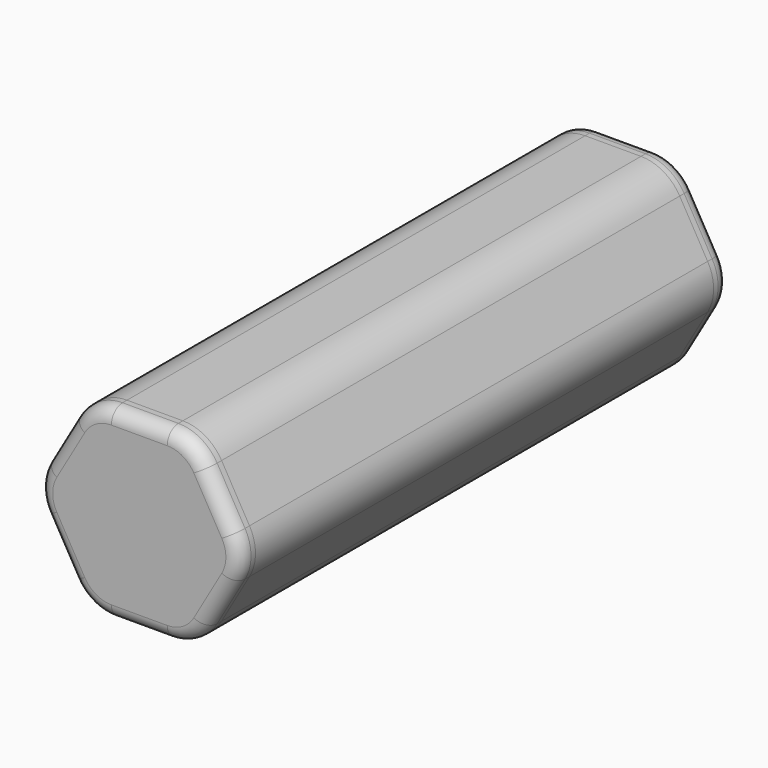
from build123d import *

# Parameters (mm, degrees)
F2_DEPTH = 205
F4_DEPTH = 5
F6_DEPTH = 2
F7_R     = 5
F8_R     = 4.99999


# Not quite as in the source:
# - a fillet or chamfer is up to 0.001 mm smaller than in the source, because OpenCascade refuses the exact size


with BuildPart() as f2:
    # F1 (on Front) → F2 (new body)
    with BuildSketch(Plane.XZ):
        with BuildLine():
            Line((30, 33.3205085668), (10, 33.3205085668))
            ThreePointArc((10, 33.3205085668), (1.9999997545, 31.1769149615), (-3.8564068859, 25.3205083212))
            Line((-3.8564068859, 25.3205083212), (-13.8564068859, 8.0000002455))
            ThreePointArc((-13.8564068859, 8.0000002455), (-16.0000004911, 0), (-13.8564068859, -8.0000002455))
            Line((-13.8564068859, -8.0000002455), (-3.8564068859, -25.3205083212))
            ThreePointArc((-3.8564068859, -25.3205083212), (1.9999997545, -31.1769149615), (10, -33.3205085668))
            Line((10, -33.3205085668), (30, -33.3205085668))
            ThreePointArc((30, -33.3205085668), (38.0000002455, -31.1769149615), (43.8564068859, -25.3205083212))
            Line((43.8564068859, -25.3205083212), (53.8564068859, -8.0000002455))
            ThreePointArc((53.8564068859, -8.0000002455), (56.0000004911, 0), (53.8564068859, 8.0000002455))
            Line((53.8564068859, 8.0000002455), (43.8564068859, 25.3205083212))
            ThreePointArc((43.8564068859, 25.3205083212), (38.0000002455, 31.1769149615), (30, 33.3205085668))
        make_face()
        with BuildLine():
            ThreePointArc((-2.1243560783, 24.3205083212), (2.9999997545, 29.444864154), (10, 31.3205085668))
            Line((10, 31.3205085668), (30, 31.3205085668))
            ThreePointArc((30, 31.3205085668), (37.0000002455, 29.444864154), (42.1243560783, 24.3205083212))
            Line((42.1243560783, 24.3205083212), (52.1243560783, 7.0000002455))
            ThreePointArc((52.1243560783, 7.0000002455), (54.0000004911, 0), (52.1243560783, -7.0000002455))
            Line((52.1243560783, -7.0000002455), (42.1243560783, -24.3205083212))
            ThreePointArc((42.1243560783, -24.3205083212), (37.0000002455, -29.444864154), (30, -31.3205085668))
            Line((30, -31.3205085668), (10, -31.3205085668))
            ThreePointArc((10, -31.3205085668), (2.9999997545, -29.444864154), (-2.1243560783, -24.3205083212))
            Line((-2.1243560783, -24.3205083212), (-12.1243560783, -7.0000002455))
            ThreePointArc((-12.1243560783, -7.0000002455), (-14.0000004911, 0), (-12.1243560783, 7.0000002455))
            Line((-12.1243560783, 7.0000002455), (-2.1243560783, 24.3205083212))
        make_face(mode=Mode.SUBTRACT)
    extrude(amount=F2_DEPTH)


with BuildPart() as f4:
    # F3 (on face) → F4 (new body)
    with BuildSketch(Plane.XZ.offset(205)):
        with BuildLine():
            ThreePointArc((-3.8564068859, -25.3205083212), (1.9999997545, -31.1769149615), (10, -33.3205085668))
            Line((10, -33.3205085668), (30, -33.3205085668))
            ThreePointArc((30, -33.3205085668), (38.0000002455, -31.1769149615), (43.8564068859, -25.3205083212))
            Line((43.8564068859, -25.3205083212), (53.8564068859, -8.0000002455))
            ThreePointArc((53.8564068859, -8.0000002455), (56.0000004911, 0), (53.8564068859, 8.0000002455))
            Line((53.8564068859, 8.0000002455), (43.8564068859, 25.3205083212))
            ThreePointArc((43.8564068859, 25.3205083212), (38.0000002455, 31.1769149615), (30, 33.3205085668))
            Line((30, 33.3205085668), (10, 33.3205085668))
            ThreePointArc((10, 33.3205085668), (1.9999997545, 31.1769149615), (-3.8564068859, 25.3205083212))
            Line((-3.8564068859, 25.3205083212), (-13.8564068859, 8.0000002455))
            ThreePointArc((-13.8564068859, 8.0000002455), (-16.0000004911, 0), (-13.8564068859, -8.0000002455))
            Line((-13.8564068859, -8.0000002455), (-3.8564068859, -25.3205083212))
        make_face()
        with BuildLine():
            ThreePointArc((-2.1243560783, 24.3205083212), (2.9999997545, 29.444864154), (10, 31.3205085668))
            Line((10, 31.3205085668), (30, 31.3205085668))
            ThreePointArc((30, 31.3205085668), (37.0000002455, 29.444864154), (42.1243560783, 24.3205083212))
            Line((42.1243560783, 24.3205083212), (52.1243560783, 7.0000002455))
            ThreePointArc((52.1243560783, 7.0000002455), (54.0000004911, 0), (52.1243560783, -7.0000002455))
            Line((52.1243560783, -7.0000002455), (42.1243560783, -24.3205083212))
            ThreePointArc((42.1243560783, -24.3205083212), (37.0000002455, -29.444864154), (30, -31.3205085668))
            Line((30, -31.3205085668), (10, -31.3205085668))
            ThreePointArc((10, -31.3205085668), (2.9999997545, -29.444864154), (-2.1243560783, -24.3205083212))
            Line((-2.1243560783, -24.3205083212), (-12.1243560783, -7.0000002455))
            ThreePointArc((-12.1243560783, -7.0000002455), (-14.0000004911, 0), (-12.1243560783, 7.0000002455))
            Line((-12.1243560783, 7.0000002455), (-2.1243560783, 24.3205083212))
        make_face(mode=Mode.SUBTRACT)
    extrude(amount=F4_DEPTH)

    # F5 (on face) → F6 (join)
    with BuildSketch(Plane.XZ.offset(210)):
        with BuildLine():
            Line((-13.8564068859, -8.0000002455), (-3.8564068859, -25.3205083212))
            ThreePointArc((-3.8564068859, -25.3205083212), (1.9999997545, -31.1769149615), (10, -33.3205085668))
            Line((10, -33.3205085668), (30, -33.3205085668))
            ThreePointArc((30, -33.3205085668), (38.0000002455, -31.1769149615), (43.8564068859, -25.3205083212))
            Line((43.8564068859, -25.3205083212), (53.8564068859, -8.0000002455))
            ThreePointArc((53.8564068859, -8.0000002455), (56.0000004911, 0), (53.8564068859, 8.0000002455))
            Line((53.8564068859, 8.0000002455), (43.8564068859, 25.3205083212))
            ThreePointArc((43.8564068859, 25.3205083212), (38.0000002455, 31.1769149615), (30, 33.3205085668))
            Line((30, 33.3205085668), (10, 33.3205085668))
            ThreePointArc((10, 33.3205085668), (1.9999997545, 31.1769149615), (-3.8564068859, 25.3205083212))
            Line((-3.8564068859, 25.3205083212), (-13.8564068859, 8.0000002455))
            ThreePointArc((-13.8564068859, 8.0000002455), (-16.0000004911, 0), (-13.8564068859, -8.0000002455))
        make_face()
        with BuildLine():
            ThreePointArc((10, -31.3205085668), (2.9999997545, -29.444864154), (-2.1243560783, -24.3205083212))
            Line((-2.1243560783, -24.3205083212), (-12.1243560783, -7.0000002455))
            ThreePointArc((-12.1243560783, -7.0000002455), (-14.0000004911, 0), (-12.1243560783, 7.0000002455))
            Line((-12.1243560783, 7.0000002455), (-2.1243560783, 24.3205083212))
            ThreePointArc((-2.1243560783, 24.3205083212), (2.9999997545, 29.444864154), (10, 31.3205085668))
            Line((10, 31.3205085668), (30, 31.3205085668))
            ThreePointArc((30, 31.3205085668), (37.0000002455, 29.444864154), (42.1243560783, 24.3205083212))
            Line((42.1243560783, 24.3205083212), (52.1243560783, 7.0000002455))
            ThreePointArc((52.1243560783, 7.0000002455), (54.0000004911, 0), (52.1243560783, -7.0000002455))
            Line((52.1243560783, -7.0000002455), (42.1243560783, -24.3205083212))
            ThreePointArc((42.1243560783, -24.3205083212), (37.0000002455, -29.444864154), (30, -31.3205085668))
            Line((30, -31.3205085668), (10, -31.3205085668))
        make_face(mode=Mode.SUBTRACT)
        with BuildLine():
            Line((-12.1243560783, -7.0000002455), (-2.1243560783, -24.3205083212))
            ThreePointArc((-2.1243560783, -24.3205083212), (2.9999997545, -29.444864154), (10, -31.3205085668))
            Line((10, -31.3205085668), (30, -31.3205085668))
            ThreePointArc((30, -31.3205085668), (37.0000002455, -29.444864154), (42.1243560783, -24.3205083212))
            Line((42.1243560783, -24.3205083212), (52.1243560783, -7.0000002455))
            ThreePointArc((52.1243560783, -7.0000002455), (54.0000004911, 0), (52.1243560783, 7.0000002455))
            Line((52.1243560783, 7.0000002455), (42.1243560783, 24.3205083212))
            ThreePointArc((42.1243560783, 24.3205083212), (37.0000002455, 29.444864154), (30, 31.3205085668))
            Line((30, 31.3205085668), (10, 31.3205085668))
            ThreePointArc((10, 31.3205085668), (2.9999997545, 29.444864154), (-2.1243560783, 24.3205083212))
            Line((-2.1243560783, 24.3205083212), (-12.1243560783, 7.0000002455))
            ThreePointArc((-12.1243560783, 7.0000002455), (-14.0000004911, 0), (-12.1243560783, -7.0000002455))
        make_face()
    extrude(amount=F6_DEPTH)

    # F7
    f7_edges = [f4.edges().sort_by_distance(p)[0] for p in [
        (-8.856407, -212, -16.660254),
        (2, -212, -31.176915),
        (20, -212, -33.320509),
        (38, -212, -31.176915),
        (48.856407, -212, -16.660254),
        (56, -212, 0),
        (48.856407, -212, 16.660254),
        (38, -212, 31.176915),
        (20, -212, 33.320509),
        (2, -212, 31.176915),
        (-8.856407, -212, 16.660254),
        (-16, -212, 0),
    ]]
    fillet(f7_edges, radius=F7_R)

    # F8 (radius 5 in the source; OpenCascade refuses exactly that, so slightly less here)
    f8_edges = [f4.edges().sort_by_distance(p)[0] for p in [
        (-7.124356, -210, -15.660254),
        (-14, -210, 0),
        (-7.124356, -210, 15.660254),
        (3, -210, 29.444864),
        (20, -210, 31.320509),
        (37, -210, 29.444864),
        (47.124356, -210, 15.660254),
        (54, -210, 0),
        (47.124356, -210, -15.660254),
        (37, -210, -29.444864),
        (20, -210, -31.320509),
        (3, -210, -29.444864),
    ]]
    fillet(f8_edges, radius=F8_R)


with BuildPart() as f10_1:
    # F10: instance of F4
    add(f4.part.mirror(Plane.XZ.offset(102.5)))


solid = Compound([f2.part, f4.part, f10_1.part])
